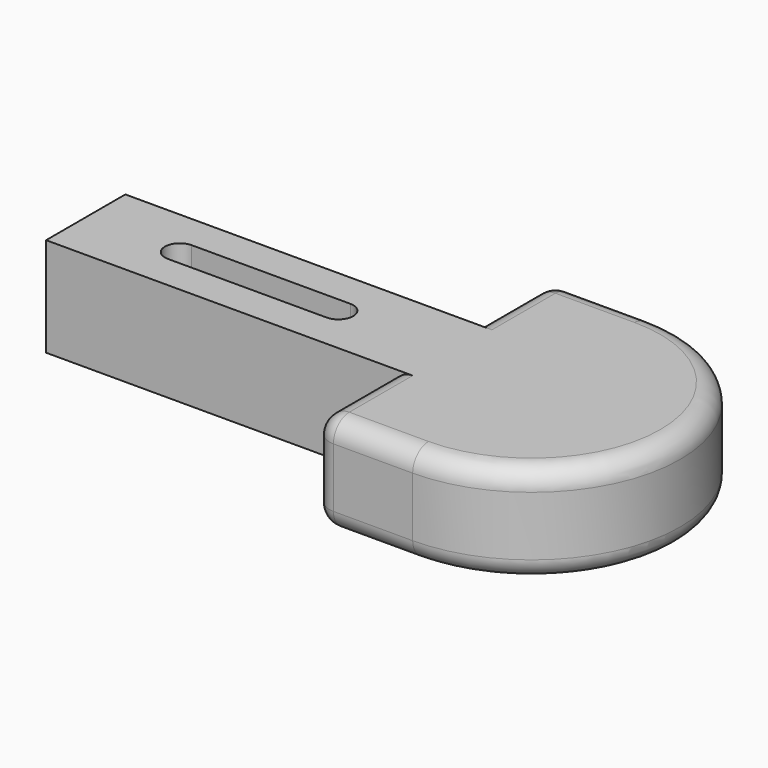
from build123d import *

# Parameters (mm, degrees)
F0_W     = 35
F0_H     = 10
F1_DEPTH = 10
F2_R     = 2


# Not quite as in the source:
# - a feature names something its author has since deleted; it is built from what else it names


with BuildPart() as f1:
    # F0 (on Top) → F1 (new body)
    with BuildSketch(Plane.XY):
        Rectangle(F0_W, F0_H)
        with BuildLine():
            Line((-8, 1.5), (0, 1.5))
            Line((0, 1.5), (8, 1.5))
            ThreePointArc((8, 1.5), (9.5, 0), (8, -1.5))
            Line((8, -1.5), (0, -1.5))
            Line((0, -1.5), (-8, -1.5))
            ThreePointArc((-8, -1.5), (-9.5, 0), (-8, 1.5))
        make_face(mode=Mode.SUBTRACT)
        Polygon((17.5, 15), (17.5, 5), (17.5, -5), (17.5, -15), (27.5, -15), (27.5, 15), align=None)
        with BuildLine():
            ThreePointArc((27.5, -15), (42.5, 0), (27.5, 15))
            Line((27.5, 15), (27.5, -15))
        make_face()
    extrude(amount=F1_DEPTH)

    # F2
    f2_edges = [f1.edges().sort_by_distance(p)[0] for p in [
        (27.5, 15, 5),
        (27.5, -15, 5),
        (42.5, 0, 10),
        (42.5, 0, 0),
        (17.5, 10, 10),
        (17.5, -10, 10),
        (17.5, -15, 5),
        (17.5, 10, 0),
        (17.5, -10, 0),
        (17.5, 15, 5),
    ]]
    fillet(f2_edges, radius=F2_R)


solid = f1.part
